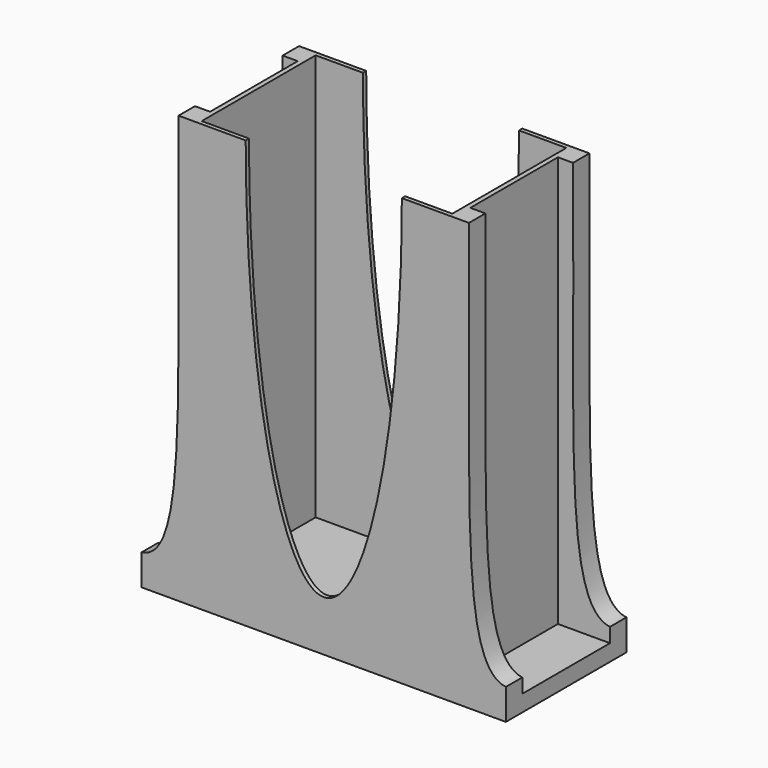
from build123d import *

# Parameters (mm, degrees)
F1_DEPTH = 27.5
F2_W     = 92
F2_H     = 160
F3_DEPTH = 26
F5_START = 20
F5_DEPTH = 7.5
F8_W     = 133
F8_H     = 6
F9_DEPTH = 27.5


# Not quite as in the source:
# - a feature names something its author has since deleted; it is built from what else it names


with BuildPart() as f1:
    # F0 (on Front) → F1 (new body, symmetric)
    with BuildSketch(Plane.XZ):
        with BuildLine():
            Line((-47.5, -75), (47.5, -75))
            Line((47.5, -75), (47.5, 75))
            Line((47.5, 75), (28.5, 75))
            add(Edge.make_bspline(
                [(0, -62.5), (28.5, -62.5), (28.5, 75)],
                knots=[0, 0, 0, 1.5707963268, 1.5707963268, 1.5707963268], degree=2, weights=[1, 0.7071067812, 1]))
            add(Edge.make_bspline(
                [(-28.5, 75), (-28.5, -62.5), (0, -62.5)],
                knots=[4.7123889804, 4.7123889804, 4.7123889804, 6.2831853072, 6.2831853072, 6.2831853072], degree=2, weights=[1, 0.7071067812, 1]))
            Line((-28.5, 75), (-47.5, 75))
            Line((-47.5, 75), (-47.5, -75))
        make_face()
    extrude(amount=F1_DEPTH, both=True)

    # F2 (on Front) → F3 (cut, symmetric)
    with BuildSketch(Plane.XZ):
        with Locations((0.2383571118, 6.4966206347)):
            Rectangle(F2_W, F2_H)
    extrude(amount=F3_DEPTH, both=True, mode=Mode.SUBTRACT)

    # F4 (on Front) → F5 (join)
    with BuildSketch(Plane.XZ.offset(F5_START)):
        with BuildLine():
            add(Edge.make_bspline(
                [(53.0086401116, 75), (53.7921645124, -12.5080782441), (49.3814773033, -67.453669192), (66.5, -69.7422416255)],
                knots=[0, 0, 0, 0, 145.3696436758, 145.3696436758, 145.3696436758, 145.3696436758], degree=3))
            Line((53.0086401116, 75), (47.5, 75))
            Line((47.5, 75), (47.5, -75))
            Line((47.5, -75), (66.5, -75))
            Line((66.5, -75), (66.5, -69.7422416255))
        make_face()
    extrude(amount=F5_DEPTH)

    # F6: F1 across plane


with BuildPart() as f1_1:
    add(f1.part)
    add(f1.part.mirror(Plane.YZ))

    # F7: F1 across plane


with BuildPart() as f1_2:
    add(f1_1.part)
    add(f1_1.part.mirror(Plane.XZ))

    # F8 (on Front) → F9 (join, symmetric)
    with BuildSketch(Plane.XZ):
        with Locations((0, -78)):
            Rectangle(F8_W, F8_H)
    extrude(amount=F9_DEPTH, both=True)


solid = f1_2.part
